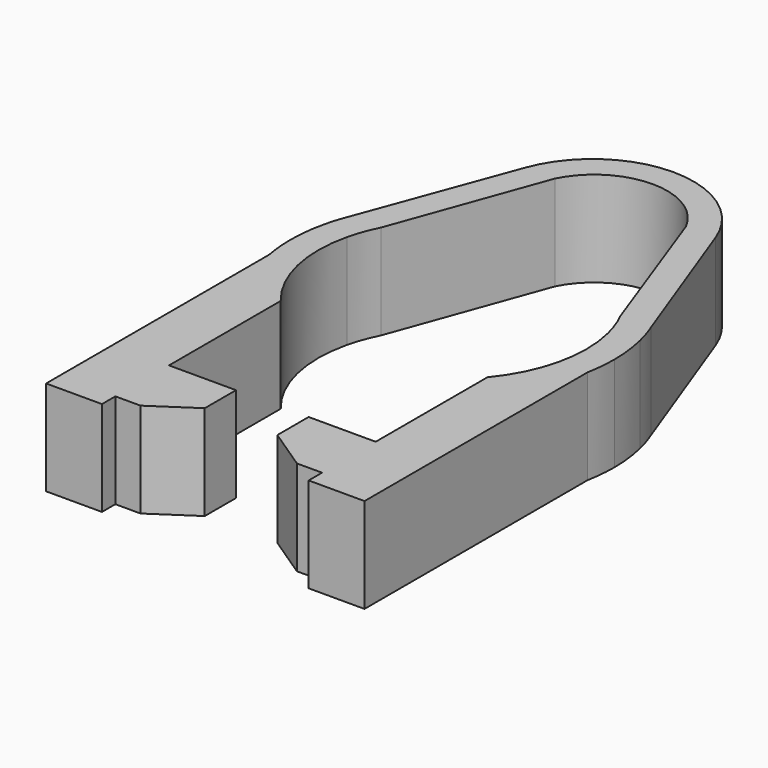
from build123d import *

# Parameters (mm, degrees)
F1_DEPTH = 8.5


# Not quite as in the source:
# - a feature names something its author has since deleted; it is built from what else it names


with BuildPart() as f1:
    # F0 (on Top) → F1 (new body)
    with BuildSketch(Plane.XY):
        with BuildLine():
            ThreePointArc((-9.25, -7.6444424257), (-11.6891485981, -2.7136331829), (-11.6717637121, 2.7874597484))
            ThreePointArc((-11.6717637121, 2.7874597484), (-11.2656904289, 4.1333060811), (-10.7050113586, 5.42242859))
            Line((-10.7050113586, 5.42242859), (-5.8459149373, 18.8072078091))
            ThreePointArc((-5.8459149373, 18.8072078091), (0, 22.4041745059), (5.8459149373, 18.8072078091))
            Line((5.8459149373, 18.8072078091), (10.7050113586, 5.42242859))
            ThreePointArc((10.7050113586, 5.42242859), (11.2656904289, 4.1333060811), (11.6717637121, 2.7874597484))
            ThreePointArc((11.6717637121, 2.7874597484), (11.6891485981, -2.7136331829), (9.25, -7.6444424257))
            Line((9.25, -7.6444424257), (9.25, -11.1663557171))
            Line((9.25, -11.1663557171), (9.25, -20.1444424257))
            Line((9.25, -20.1444424257), (3.25, -20.1444424257))
            Line((3.25, -20.1444424257), (3.25, -21.1444424257))
            Line((3.25, -21.1444424257), (3.25, -23.6444424257))
            Line((3.25, -23.6444424257), (7, -26.1444424257))
            Line((7, -26.1444424257), (9.25, -26.1444424257))
            Line((9.25, -26.1444424257), (9.25, -27.6444424257))
            Line((9.25, -27.6444424257), (14.25, -27.6444424257))
            Line((14.25, -27.6444424257), (14.25, -21.4303609628))
            Line((14.25, -21.4303609628), (14.25, -2.6809513237))
            ThreePointArc((14.25, -2.6809513237), (14.437364718, -1.3462912018), (14.5, 0))
            ThreePointArc((14.5, 0), (14.400503927, 1.6957259941), (14.1033811521, 3.3681805293))
            ThreePointArc((14.1033811521, 3.3681805293), (13.8091695526, 4.4223111907), (13.4362898945, 5.4512488358))
            Line((13.4362898945, 5.4512488358), (8.4985279846, 18.8072078091))
            ThreePointArc((8.4985279846, 18.8072078091), (0, 24.7259901099), (-8.4985279846, 18.8072078091))
            Line((-8.4985279846, 18.8072078091), (-13.4362898945, 5.4512488358))
            ThreePointArc((-13.4362898945, 5.4512488358), (-13.8091695526, 4.4223111907), (-14.1033811521, 3.3681805293))
            ThreePointArc((-14.1033811521, 3.3681805293), (-14.400503927, 1.6957259941), (-14.5, 0))
            ThreePointArc((-14.5, 0), (-14.437364718, -1.3462912018), (-14.25, -2.6809513237))
            Line((-14.25, -2.6809513237), (-14.25, -21.1444424257))
            Line((-14.25, -21.1444424257), (-14.25, -27.6444424257))
            Line((-14.25, -27.6444424257), (-9.25, -27.6444424257))
            Line((-9.25, -27.6444424257), (-9.25, -26.1444424257))
            Line((-9.25, -26.1444424257), (-7, -26.1444424257))
            Line((-7, -26.1444424257), (-3.25, -23.6444424257))
            Line((-3.25, -23.6444424257), (-3.25, -21.1444424257))
            Line((-3.25, -21.1444424257), (-3.25, -20.1444424257))
            Line((-3.25, -20.1444424257), (-9.25, -20.1444424257))
            Line((-9.25, -20.1444424257), (-9.25, -11.1663557171))
            Line((-9.25, -11.1663557171), (-9.25, -7.6444424257))
        make_face()
    extrude(amount=-F1_DEPTH)


solid = f1.part
